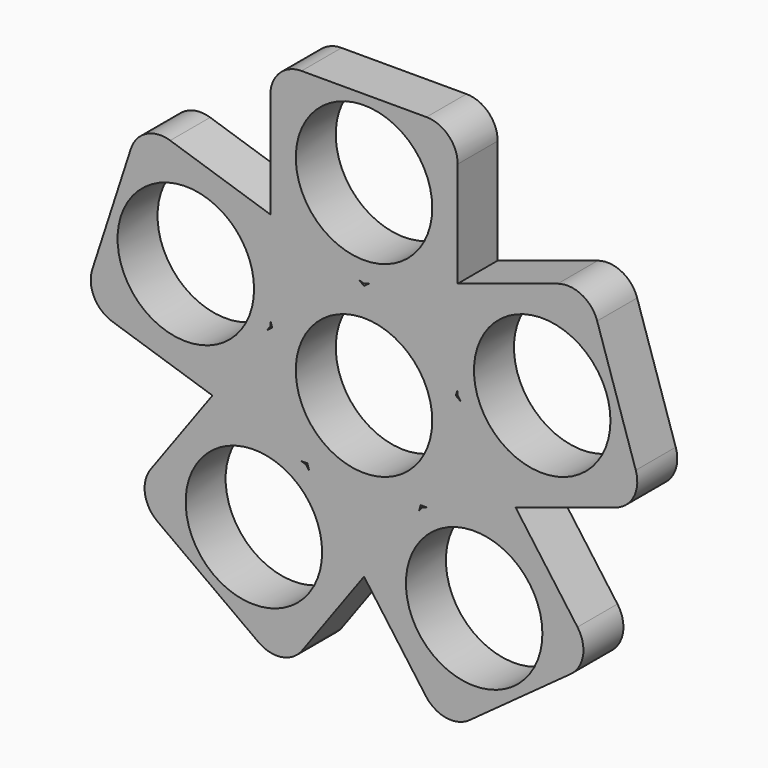
from build123d import *

# Parameters (mm, degrees)
F0_R     = 10.925
F1_DEPTH = 8


with BuildPart() as f1:
    # F0 (on Front) → F1 (new body)
    with BuildSketch(Plane.XZ):
        Polygon((137.5925300597, 43.0939033628), (138.203267445, 43.0939033628), (132.6625055075, 50.7201079193), (132.6625055075, 44.6957654427), align=None)
        Polygon((132.6625055075, 66.4920412828), (138.3919956762, 68.353665488), (141.9330153387, 73.2274609315), (132.6625055075, 76.2396321698), align=None)
        with BuildLine():
            Line((152.4504447694, 74.5233945768), (153.3919956762, 73.2274609315))
            Line((153.3919956762, 73.2274609315), (162.6625055075, 76.2396321698))
            Line((162.6625055075, 76.2396321698), (162.6625055075, 93.0939033628))
            ThreePointArc((162.6625055075, 93.0939033628), (161.1980394134, 96.6294372687), (157.6625055075, 98.0939033628))
            Line((157.6625055075, 98.0939033628), (137.6625055075, 98.0939033628))
            ThreePointArc((137.6625055075, 98.0939033628), (134.1269716015, 96.6294372687), (132.6625055075, 93.0939033628))
            Line((132.6625055075, 93.0939033628), (132.6625055075, 76.2396321698))
            Line((132.6625055075, 76.2396321698), (141.9330153387, 73.2274609315))
            Line((141.9330153387, 73.2274609315), (142.8745662455, 74.5233945768))
            Line((142.8745662455, 74.5233945768), (146.8630398909, 71.6255988516))
            Line((146.8630398909, 71.6255988516), (147.6625055075, 71.3658367263))
            Line((147.6625055075, 71.3658367263), (148.461971124, 71.6255988516))
            Line((148.461971124, 71.6255988516), (152.4504447694, 74.5233945768))
        make_face()
        with Locations((147.6625055075, 85.5939033628)):
            Circle(F0_R, mode=Mode.SUBTRACT)
        Polygon((153.3919956762, 73.2274609315), (156.9330153387, 68.353665488), (162.6625055075, 66.4920412828), (162.6625055075, 76.2396321698), align=None)
        Polygon((147.9678742002, 71.2666164235), (156.9330153387, 68.353665488), (153.3919956762, 73.2274609315), (148.461971124, 71.6255988516), align=None)
        Polygon((138.5807239074, 43.0939033628), (156.7442871075, 43.0939033628), (162.3571368148, 60.3684785034), (147.6625055075, 71.0447530815), (132.9678742002, 60.3684785034), align=None)
        with Locations((147.6625055075, 55.5939033628)):
            Circle(F0_R, mode=Mode.SUBTRACT)
        Polygon((147.6625055075, 30.0743791122), (153.3919956762, 37.960345794), (147.6625055075, 39.8219699992), (141.9330153387, 37.960345794), align=None)
        with BuildLine():
            Line((137.7558134621, 16.4389872893), (147.6625055075, 30.0743791122))
            Line((147.6625055075, 30.0743791122), (141.9330153387, 37.960345794))
            Line((141.9330153387, 37.960345794), (140.4095539694, 37.4653431886))
            Line((140.4095539694, 37.4653431886), (138.8860926001, 42.1540751645))
            Line((138.8860926001, 42.1540751645), (138.3919956762, 42.8341412375))
            Line((138.3919956762, 42.8341412375), (137.5925300597, 43.0939033628))
            Line((137.5925300597, 43.0939033628), (132.6625055075, 43.0939033628))
            Line((132.6625055075, 43.0939033628), (132.6625055075, 44.6957654427))
            Line((132.6625055075, 44.6957654427), (123.3919956762, 47.707936681))
            Line((123.3919956762, 47.707936681), (113.4853036309, 34.0725448581))
            ThreePointArc((113.4853036309, 34.0725448581), (112.5919468998, 30.3514462714), (114.5914623413, 27.0885336247))
            Line((114.5914623413, 27.0885336247), (130.7718022288, 15.3328285789))
            ThreePointArc((130.7718022288, 15.3328285789), (134.4929008155, 14.4394718478), (137.7558134621, 16.4389872893))
        make_face()
        with Locations((130.0289479387, 31.3233935315)):
            Circle(F0_R, mode=Mode.SUBTRACT)
        with BuildLine():
            Line((162.6625055075, 44.6957654427), (162.6625055075, 43.0939033628))
            Line((162.6625055075, 43.0939033628), (157.7324809553, 43.0939033628))
            Line((157.7324809553, 43.0939033628), (156.9330153387, 42.8341412375))
            Line((156.9330153387, 42.8341412375), (156.4389184148, 42.1540751645))
            Line((156.4389184148, 42.1540751645), (154.9154570455, 37.4653431886))
            Line((154.9154570455, 37.4653431886), (153.3919956762, 37.960345794))
            Line((153.3919956762, 37.960345794), (147.6625055075, 30.0743791122))
            Line((147.6625055075, 30.0743791122), (157.5691975528, 16.4389872893))
            ThreePointArc((157.5691975528, 16.4389872893), (160.8321101995, 14.4394718478), (164.5532087862, 15.3328285789))
            Line((164.5532087861, 15.3328285789), (180.7335486736, 27.0885336247))
            ThreePointArc((180.7335486736, 27.0885336247), (182.7330641152, 30.3514462714), (181.8397073841, 34.0725448581))
            Line((181.8397073841, 34.0725448581), (171.9330153387, 47.707936681))
            Line((171.9330153387, 47.707936681), (162.6625055075, 44.6957654427))
        make_face()
        with Locations((165.2960630762, 31.3233935315)):
            Circle(F0_R, mode=Mode.SUBTRACT)
        with BuildLine():
            Line((166.20352517, 55.5939033628), (171.9330153387, 47.707936681))
            Line((171.9330153387, 47.707936681), (187.9623797842, 52.9161929074))
            ThreePointArc((187.9623797842, 52.9161929074), (190.8723274332, 55.4015229902), (191.1725773938, 59.2165604607))
            Line((191.1725773938, 59.2165604607), (184.9922375063, 78.2376907866))
            ThreePointArc((184.9922375063, 78.2376907866), (182.5069074235, 81.1476384357), (178.6918699529, 81.4478883962))
            Line((178.6918699529, 81.4478883962), (162.6625055075, 76.2396321698))
            Line((162.6625055075, 76.2396321698), (162.6625055075, 66.4920412828))
            Line((162.6625055075, 66.4920412828), (164.1859668768, 65.9970386775))
            Line((164.1859668768, 65.9970386775), (162.6625055075, 61.3083067016))
            Line((162.6625055075, 61.3083067016), (162.6625055075, 60.4676988062))
            Line((162.6625055075, 60.4676988062), (163.1566024313, 59.7876327333))
            Line((163.1566024313, 59.7876327333), (167.1450760767, 56.8898370081))
            Line((167.1450760767, 56.8898370081), (166.20352517, 55.5939033628))
        make_face()
        with Locations((176.1942009963, 64.864413194)):
            Circle(F0_R, mode=Mode.SUBTRACT)
        Polygon((162.6625055075, 50.7201079193), (162.6625055075, 44.6957654427), (171.9330153387, 47.707936681), (166.20352517, 55.5939033628), align=None)
        Polygon((162.6625055075, 60.1466151614), (162.6625055075, 50.7201079193), (166.20352517, 55.5939033628), (163.1566024313, 59.7876327333), align=None)
        Polygon((163.1566024313, 59.7876327333), (166.20352517, 55.5939033628), (167.1450760767, 56.8898370081), align=None)
        Polygon((156.7442871075, 43.0939033628), (157.1217435699, 43.0939033628), (162.6625055075, 50.7201079193), (162.6625055075, 60.1466151614), (162.3571368148, 60.3684785034), align=None)
        Polygon((157.1217435699, 43.0939033628), (157.7324809553, 43.0939033628), (162.6625055075, 44.6957654427), (162.6625055075, 50.7201079193), align=None)
        Polygon((157.7324809553, 43.0939033628), (162.6625055075, 43.0939033628), (162.6625055075, 44.6957654427), align=None)
        Polygon((154.9154570455, 37.4653431886), (156.4389184148, 42.1540751645), (153.3919956762, 37.960345794), align=None)
        Polygon((153.3919956762, 37.960345794), (156.4389184148, 42.1540751645), (156.627646646, 42.7349209346), (147.6625055075, 39.8219699992), align=None)
        Polygon((156.627646646, 42.7349209346), (156.7442871075, 43.0939033628), (138.5807239074, 43.0939033628), (138.6973643689, 42.7349209346), (147.6625055075, 39.8219699992), align=None)
        Polygon((141.9330153387, 37.960345794), (147.6625055075, 39.8219699992), (138.6973643689, 42.7349209346), (138.8860926001, 42.1540751645), align=None)
        Polygon((140.4095539694, 37.4653431886), (141.9330153387, 37.960345794), (138.8860926001, 42.1540751645), align=None)
        Polygon((138.203267445, 43.0939033628), (138.5807239074, 43.0939033628), (132.9678742002, 60.3684785034), (132.6625055075, 60.1466151614), (132.6625055075, 50.7201079193), align=None)
        Polygon((132.6625055075, 43.0939033628), (137.5925300597, 43.0939033628), (132.6625055075, 44.6957654427), align=None)
        Polygon((132.6625055075, 44.6957654427), (132.6625055075, 50.7201079193), (129.121485845, 55.5939033628), (123.3919956762, 47.707936681), align=None)
        Polygon((129.121485845, 55.5939033628), (132.6625055075, 50.7201079193), (132.6625055075, 60.1466151614), (132.1684085836, 59.7876327333), align=None)
        Polygon((128.1799349382, 56.8898370081), (129.121485845, 55.5939033628), (132.1684085836, 59.7876327333), align=None)
        Polygon((132.6625055075, 61.3083067016), (132.8512337387, 60.7274609315), (138.3919956762, 68.353665488), (132.6625055075, 66.4920412828), align=None)
        Polygon((131.1390441382, 65.9970386775), (132.6625055075, 61.3083067016), (132.6625055075, 66.4920412828), align=None)
        Polygon((132.8512337387, 60.7274609315), (132.9678742002, 60.3684785034), (147.6625055075, 71.0447530815), (147.3571368148, 71.2666164235), (138.3919956762, 68.353665488), align=None)
        Polygon((141.9330153387, 73.2274609315), (146.8630398909, 71.6255988516), (142.8745662455, 74.5233945768), align=None)
        Polygon((138.3919956762, 68.353665488), (147.3571368148, 71.2666164235), (146.8630398909, 71.6255988516), (141.9330153387, 73.2274609315), align=None)
        Polygon((147.6625055075, 71.0447530815), (162.3571368148, 60.3684785034), (162.4737772763, 60.7274609315), (156.9330153387, 68.353665488), (147.9678742002, 71.2666164235), align=None)
        Polygon((156.9330153387, 68.353665488), (162.4737772763, 60.7274609315), (162.6625055075, 61.3083067016), (162.6625055075, 66.4920412828), align=None)
        Polygon((162.6625055075, 66.4920412828), (162.6625055075, 61.3083067016), (164.1859668768, 65.9970386775), align=None)
        Polygon((148.461971124, 71.6255988516), (153.3919956762, 73.2274609315), (152.4504447694, 74.5233945768), align=None)
        with BuildLine():
            Line((123.3919956762, 47.707936681), (129.121485845, 55.5939033628))
            Line((129.121485845, 55.5939033628), (128.1799349382, 56.8898370081))
            Line((128.1799349382, 56.8898370081), (132.1684085836, 59.7876327333))
            Line((132.1684085836, 59.7876327333), (132.6625055075, 60.4676988062))
            Line((132.6625055075, 60.4676988062), (132.6625055075, 61.3083067016))
            Line((132.6625055075, 61.3083067016), (131.1390441382, 65.9970386775))
            Line((131.1390441382, 65.9970386775), (132.6625055075, 66.4920412828))
            Line((132.6625055075, 66.4920412828), (132.6625055075, 76.2396321698))
            Line((132.6625055075, 76.2396321698), (116.633141062, 81.4478883962))
            ThreePointArc((116.633141062, 81.4478883962), (112.8181035915, 81.1476384357), (110.3327735087, 78.2376907866))
            Line((110.3327735087, 78.2376907866), (104.1524336212, 59.2165604607))
            ThreePointArc((104.1524336212, 59.2165604607), (104.4526835817, 55.4015229902), (107.3626312308, 52.9161929074))
            Line((107.3626312308, 52.9161929074), (123.3919956762, 47.707936681))
        make_face()
        with Locations((119.1308100186, 64.864413194)):
            Circle(F0_R, mode=Mode.SUBTRACT)
    extrude(amount=F1_DEPTH)


solid = f1.part
